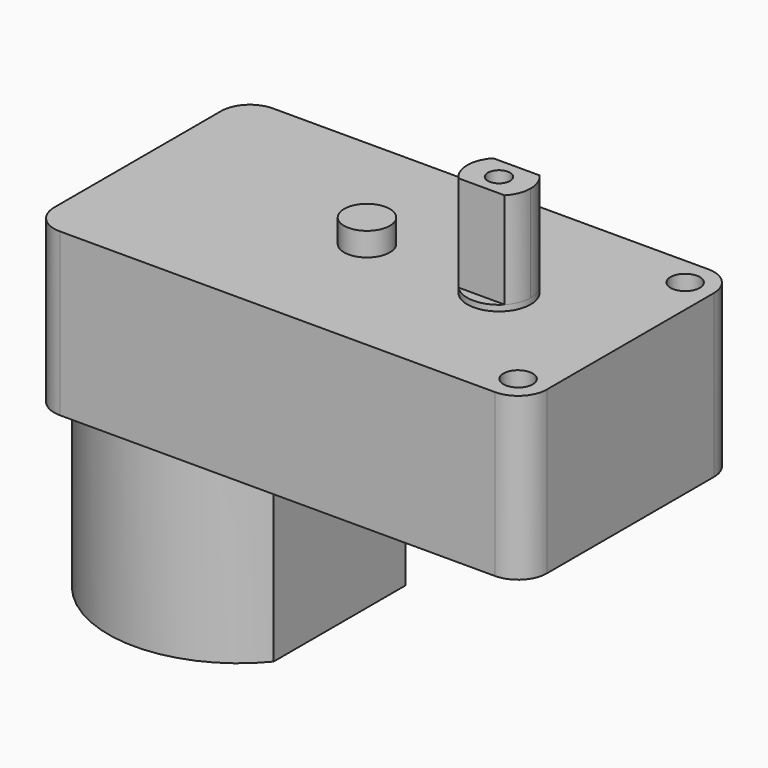
from build123d import *

# Parameters (mm, degrees)
F0_R      = 1.25
F0_R_2    = 2.7
F1_DEPTH  = 6.9
F0_R_3    = 0.95
F2_DEPTH  = 6.9
F3_DEPTH  = 7.4
F4_R      = 0.95
F5_DEPTH  = 8.2
F6_DEPTH  = 6.9
F9_DEPTH  = 15.45
F10_DEPTH = 1.5
F8_R      = 1
F11_DEPTH = 5.2
F12_R     = 1.95
F13_DEPTH = 2


with BuildPart() as f1:
    # F0 (on Top) → F1 (new body, symmetric)
    with BuildSketch(Plane.XY):
        with BuildLine():
            ThreePointArc((21, 8.9), (20.2824116139, 10.6324116139), (18.55, 11.35))
            Line((18.55, 11.35), (-18.55, 11.35))
            ThreePointArc((-18.55, 11.35), (-20.2824116139, 10.6324116139), (-21, 8.9))
            Line((-21, 8.9), (-21, -8.9))
            ThreePointArc((-21, -8.9), (-20.2824116139, -10.6324116139), (-18.55, -11.35))
            Line((-18.55, -11.35), (18.55, -11.35))
            ThreePointArc((18.55, -11.35), (20.2824116139, -10.6324116139), (21, -8.9))
            Line((21, -8.9), (21, 8.9))
        make_face()
        with Locations((18.55, -8.9)):
            Circle(F0_R, mode=Mode.SUBTRACT)
        with Locations((9.8, 0)):
            Circle(F0_R_2, mode=Mode.SUBTRACT)
        with Locations((18.55, 8.9)):
            Circle(F0_R, mode=Mode.SUBTRACT)
    extrude(amount=F1_DEPTH, both=True)

    # F0 (on Top) → F6 (join, through all)
    with BuildSketch(Plane.XY):
        with Locations((9.8, 0)):
            Circle(F0_R_2)
        with Locations((9.8, 0)):
            Circle(F0_R_3, mode=Mode.SUBTRACT)
        with Locations((9.8, 0)):
            Circle(F0_R_3)
    extrude(amount=-F6_DEPTH)

    # F7: union 

    # F8 (on face) → F9 (join)
    with BuildSketch(Plane(origin=(0, 0, -6.9), x_dir=(1, 0, 0), z_dir=(0, 0, -1))):
        with BuildLine():
            ThreePointArc((-3.8, 7.0178344238), (-12.4, 11.1), (-21, 7.0178344238))
            Line((-21, 7.0178344238), (-21, 2.1))
            Line((-21, 2.1), (-21, -2.1))
            Line((-21, -2.1), (-21, -7.0178344238))
            ThreePointArc((-21, -7.0178344238), (-12.4, -11.1), (-3.8, -7.0178344238))
            Line((-3.8, -7.0178344238), (-3.8, -2.1))
            Line((-3.8, -2.1), (-3.8, 2.1))
            Line((-3.8, 2.1), (-3.8, 7.0178344238))
        make_face()
        with BuildLine():
            ThreePointArc((-20, 6.6520673478), (-12.4, 10.1), (-4.8, 6.6520673478))
            Line((-4.8, 6.6520673478), (-4.8, -6.6520673478))
            ThreePointArc((-4.8, -6.6520673478), (-12.4, -10.1), (-20, -6.6520673478))
            Line((-20, -6.6520673478), (-20, 6.6520673478))
        make_face(mode=Mode.SUBTRACT)
    extrude(amount=F9_DEPTH)

    # F8 (on face) → F10 (join)
    with BuildSketch(Plane(origin=(0, 0, -6.9), x_dir=(1, 0, 0), z_dir=(0, 0, -1))):
        with BuildLine():
            Line((-21, -2.1), (-21, 2.1))
            Line((-21, 2.1), (-24.2, 2.1))
            ThreePointArc((-24.2, 2.1), (-22.7150757595, 1.4849242405), (-22.1, 0))
            ThreePointArc((-22.1, 0), (-22.7150757595, -1.4849242405), (-24.2, -2.1))
            Line((-24.2, -2.1), (-21, -2.1))
        make_face()
    extrude(amount=F10_DEPTH)

    # F8 (on face) → F11 (join)
    with BuildSketch(Plane(origin=(0, 0, -6.9), x_dir=(1, 0, 0), z_dir=(0, 0, -1))):
        with BuildLine():
            ThreePointArc((-22.1, 0), (-22.7150757595, 1.4849242405), (-24.2, 2.1))
            ThreePointArc((-24.2, 2.1), (-25.6849242405, 1.4849242405), (-26.3, 0))
            ThreePointArc((-26.3, 0), (-25.6849242405, -1.4849242405), (-24.2, -2.1))
            ThreePointArc((-24.2, -2.1), (-22.7150757595, -1.4849242405), (-22.1, 0))
        make_face()
        with Locations((-24.2, 0)):
            Circle(F8_R, mode=Mode.SUBTRACT)
        with BuildLine():
            ThreePointArc((1.5, 0), (0.8849242405, 1.4849242405), (-0.6, 2.1))
            ThreePointArc((-0.6, 2.1), (-2.7, 0), (-0.6, -2.1))
            ThreePointArc((-0.6, -2.1), (0.8849242405, -1.4849242405), (1.5, 0))
        make_face()
        with Locations((-0.6, 0)):
            Circle(F8_R, mode=Mode.SUBTRACT)
    extrude(amount=F11_DEPTH)

    # F12 (on face) → F13 (join)
    with BuildSketch(Plane.XY.offset(6.9)):
        with Locations((-1.45, 0)):
            Circle(F12_R)
    extrude(amount=F13_DEPTH)


with BuildPart() as f2:
    # F0 (on Top) → F2 (new body)
    with BuildSketch(Plane.XY):
        with Locations((9.8, 0)):
            Circle(F0_R_3)
    extrude(amount=F2_DEPTH)

    # F0 (on Top) → F3 (join)
    with BuildSketch(Plane.XY):
        with Locations((9.8, 0)):
            Circle(F0_R_2)
        with Locations((9.8, 0)):
            Circle(F0_R_3, mode=Mode.SUBTRACT)
    extrude(amount=F3_DEPTH)

    # F4 (on face) → F5 (join)
    with BuildSketch(Plane.XY.offset(7.4)):
        with BuildLine():
            ThreePointArc((11.7665960439, -1.85), (12.3099610872, -0.9950353465), (12.5, 0))
            ThreePointArc((12.5, 0), (12.3099610872, 0.9950353465), (11.7665960439, 1.85))
            Line((11.7665960439, 1.85), (7.8334039561, 1.85))
            ThreePointArc((7.8334039561, 1.85), (7.1, 0), (7.8334039561, -1.85))
            Line((7.8334039561, -1.85), (11.7665960439, -1.85))
        make_face()
        with Locations((9.8, 0)):
            Circle(F4_R, mode=Mode.SUBTRACT)
    extrude(amount=F5_DEPTH)


solid = Compound([f1.part, f2.part])
